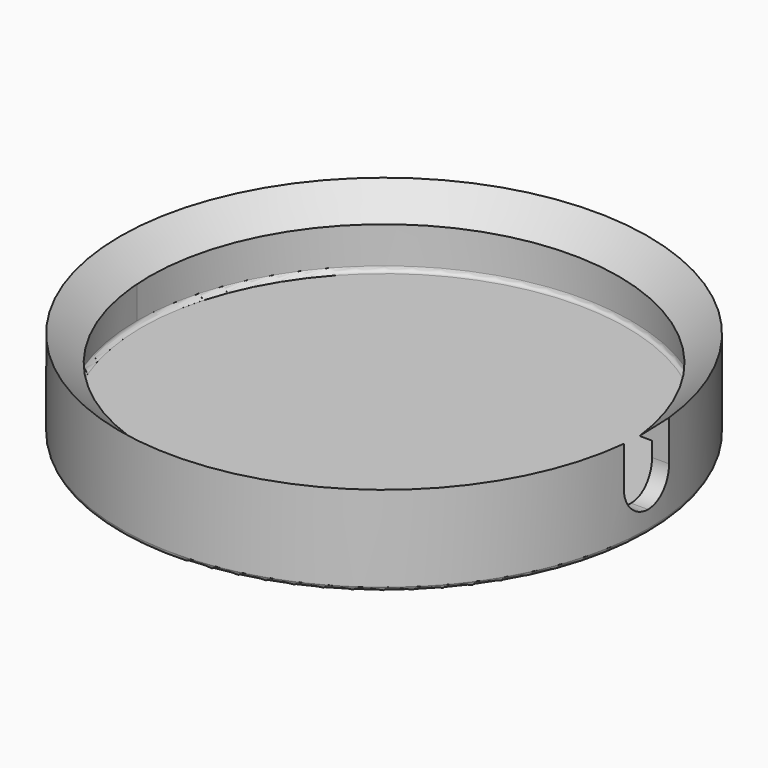
from build123d import *

# Parameters (mm, degrees)
F0_R     = 29.718
F1_DEPTH = 10.16
F6_R     = 0.508
F8_W     = 4.7481491719
F8_H     = 6.35
F9_DEPTH = 25.4
F10_R    = 3.17499


# Not quite as in the source:
# - a fillet or chamfer is up to 0.001 mm smaller than in the source, because OpenCascade refuses the exact size


with BuildPart() as f1:
    # F0 (on Top) → F1 (new body)
    with BuildSketch(Plane.XY):
        Circle(F0_R)
    extrude(amount=F1_DEPTH)

    # F2 (on Front) → F3 (revolve, cut)
    with BuildSketch(Plane.XZ):
        Polygon((29.718, 10.16), (0, 10.16), (0, 7.2644), (26.416, 7.2644), align=None)
    revolve(axis=Axis((0, 0, 8.7122), (0, 0, 1)), mode=Mode.SUBTRACT)

    # F4 (on Front) → F5 (revolve, cut)
    with BuildSketch(Plane.XZ):
        Polygon((0, 7.2644), (-26.416, 7.2644), (-27.813, 7.2644), (-27.813, 1.905), (0, 1.905), align=None)
    revolve(axis=Axis((0, 0, 4.5847), (0, 0, 1)), mode=Mode.SUBTRACT)

    # F6
    f6_edges = [f1.edges().sort_by_distance(p)[0] for p in [
        (27.813, 0, 1.905),
        (-29.718, 0, 0),
    ]]
    fillet(f6_edges, radius=F6_R)

    # F8 (on face) → F9 (cut)
    with BuildSketch(Plane.XY.offset(2.413)):
        with Locations((28.1168716028, 0)):
            Rectangle(F8_W, F8_H)
    extrude(amount=F9_DEPTH, mode=Mode.SUBTRACT)

    # F10 (radius 3.175 in the source; OpenCascade refuses exactly that, so slightly less here)
    f10_edges = [f1.edges().sort_by_distance(p)[0] for p in [
        (28.589546, 3.175, 2.413),
        (28.589546, -3.175, 2.413),
    ]]
    fillet(f10_edges, radius=F10_R)


solid = f1.part
